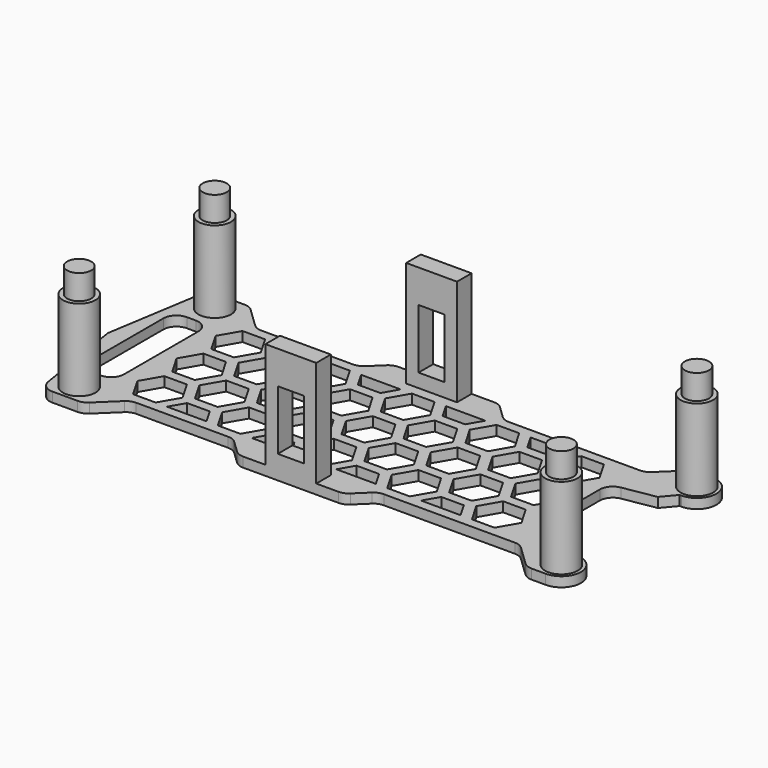
from build123d import *

# Parameters (mm, degrees)
F0_R         = 2.5
F0_W         = 5.3888335824
F0_H         = 18.2664785534
F1_DEPTH     = 1.5
F0_R_2       = 1.85
F2_DEPTH     = 14
F0_W_2       = 7.8
F0_H_2       = 2.8
F3_DEPTH     = 17.8
F4_W         = 3.9957887493
F4_H         = 9.1363643296
F5_DEPTH     = 32
F6_T4_DEPTH  = 11.8090227147
F6_S5_R      = 3
F6_T6_DEPTH  = 8
F6_T10_DEPTH = 11.8090227147
F6_S11_R     = 3
F6_T12_DEPTH = 8
F7_R         = 2


# Not quite as in the source:
# - a fillet or chamfer that OpenCascade refuses, or shapes differently, is made with other operations: its cross-section is extruded or revolved along the edge and cut away or added


with BuildPart() as f1:
    # F0 (on Top) → F1 (new body)
    with BuildSketch(Plane.XY):
        with BuildLine():
            Line((40, 8.2992520183), (40, 10))
            ThreePointArc((40, 10), (43, 13), (40, 16))
            Line((40, 16), (37.0306753963, 16))
            Line((37.0306753963, 16), (32.8572866916, 12))
            Line((32.8572866916, 12), (11.1427133083, 12))
            Line((11.1427133083, 12), (8.1170064975, 14.9))
            Line((8.1170064975, 14.9), (3.9, 14.9))
            Line((3.9, 14.9), (3.9, 12.1))
            Line((3.9, 12.1), (-3.9, 12.1))
            Line((-3.9, 12.1), (-3.9, 14.9))
            Line((-3.9, 14.9), (-8.1170064975, 14.9))
            Line((-8.1170064975, 14.9), (-11.1427133083, 12))
            Line((-11.1427133083, 12), (-26.8572866917, 12))
            Line((-26.8572866917, 12), (-31.0306753963, 16))
            Line((-31.0306753963, 16), (-37.4269299209, 16))
            Line((-37.4269299209, 16), (-40, 0))
            Line((-40, 0), (-37.4269299209, -16))
            Line((-37.4269299209, -16), (-31.0306753963, -16))
            Line((-31.0306753963, -16), (-26.8572866917, -12))
            Line((-26.8572866917, -12), (-11.1427133083, -12))
            Line((-11.1427133083, -12), (-8.1170064975, -14.9))
            Line((-8.1170064975, -14.9), (-3.9, -14.9))
            Line((-3.9, -14.9), (-3.9, -12.1))
            Line((-3.9, -12.1), (3.9, -12.1))
            Line((3.9, -12.1), (3.9, -14.9))
            Line((3.9, -14.9), (8.1170064975, -14.9))
            Line((8.1170064975, -14.9), (11.1427133083, -12))
            Line((11.1427133083, -12), (32.8572866916, -12))
            Line((32.8572866916, -12), (37.0306753963, -16))
            Line((37.0306753963, -16), (40, -16))
            ThreePointArc((40, -16), (43, -13), (40, -10))
            Line((40, -10), (40, -8.2992520183))
            Line((40, -8.2992520183), (31.389541924, -6.8237371743))
            Line((31.389541924, -6.8237371743), (31.389541924, 0))
            Line((31.389541924, 0), (31.389541924, 6.8237371743))
            Line((31.389541924, 6.8237371743), (40, 8.2992520183))
        make_face()
        with Locations((-34, -13)):
            Circle(F0_R, mode=Mode.SUBTRACT)
        Polygon((-16.4689110868, -10.5), (-22.5310889132, -10.5), (-21.2320508076, -8.25), (-17.7679491924, -8.25), align=None, mode=Mode.SUBTRACT)
        Polygon((-8.2320508076, -8.25), (-4.7679491924, -8.25), (-3.4689110868, -10.5), (-9.5310889132, -10.5), align=None, mode=Mode.SUBTRACT)
        Polygon((-24.2679491924, -10.5), (-27.7320508076, -10.5), (-29.4641016151, -7.5), (-27.7320508076, -4.5), (-24.2679491924, -4.5), (-22.5358983849, -7.5), align=None, mode=Mode.SUBTRACT)
        Polygon((-22.9641016151, -3.75), (-21.2320508076, -0.75), (-17.7679491924, -0.75), (-16.0358983849, -3.75), (-17.7679491924, -6.75), (-21.2320508076, -6.75), align=None, mode=Mode.SUBTRACT)
        Polygon((-11.2679491924, -10.5), (-14.7320508076, -10.5), (-16.4641016151, -7.5), (-14.7320508076, -4.5), (-11.2679491924, -4.5), (-9.5358983849, -7.5), align=None, mode=Mode.SUBTRACT)
        Polygon((-3.4641016151, -7.5), (-1.7320508076, -4.5), (1.7320508076, -4.5), (3.4641016151, -7.5), (1.7320508076, -10.5), (-1.7320508076, -10.5), align=None, mode=Mode.SUBTRACT)
        Polygon((-9.9641016151, -3.75), (-8.2320508076, -0.75), (-4.7679491924, -0.75), (-3.0358983849, -3.75), (-4.7679491924, -6.75), (-8.2320508076, -6.75), align=None, mode=Mode.SUBTRACT)
        Polygon((4.7679491924, -8.25), (8.2320508076, -8.25), (9.5310889132, -10.5), (3.4689110868, -10.5), align=None, mode=Mode.SUBTRACT)
        Polygon((17.7679491924, -8.25), (21.2320508076, -8.25), (22.5310889132, -10.5), (16.4689110868, -10.5), align=None, mode=Mode.SUBTRACT)
        with Locations((40, -13)):
            Circle(F0_R, mode=Mode.SUBTRACT)
        Polygon((11.2679491924, -10.5), (9.5358983849, -7.5), (11.2679491924, -4.5), (14.7320508076, -4.5), (16.4641016151, -7.5), (14.7320508076, -10.5), align=None, mode=Mode.SUBTRACT)
        Polygon((8.2320508076, -0.75), (9.9641016151, -3.75), (8.2320508076, -6.75), (4.7679491924, -6.75), (3.0358983849, -3.75), (4.7679491924, -0.75), align=None, mode=Mode.SUBTRACT)
        Polygon((16.0358983849, -3.75), (17.7679491924, -0.75), (21.2320508076, -0.75), (22.9641016151, -3.75), (21.2320508076, -6.75), (17.7679491924, -6.75), align=None, mode=Mode.SUBTRACT)
        Polygon((24.2679491924, -10.5), (22.5358983849, -7.5), (24.2679491924, -4.5), (27.7320508076, -4.5), (29.4641016151, -7.5), (27.7320508076, -10.5), align=None, mode=Mode.SUBTRACT)
        with Locations((-34.495420754, 0)):
            Rectangle(F0_W, F0_H, mode=Mode.SUBTRACT)
        Polygon((-27.7320508076, -3), (-29.4641016151, 0), (-27.7320508076, 3), (-24.2679491924, 3), (-22.5358983849, 0), (-24.2679491924, -3), align=None, mode=Mode.SUBTRACT)
        Polygon((-17.7679491924, 6.75), (-16.0358983849, 3.75), (-17.7679491924, 0.75), (-21.2320508076, 0.75), (-22.9641016151, 3.75), (-21.2320508076, 6.75), align=None, mode=Mode.SUBTRACT)
        Polygon((-29.4641016151, 7.5), (-27.7320508076, 10.5), (-24.2679491924, 10.5), (-22.5358983849, 7.5), (-24.2679491924, 4.5), (-27.7320508076, 4.5), align=None, mode=Mode.SUBTRACT)
        Polygon((-14.7320508076, -3), (-16.4641016151, 0), (-14.7320508076, 3), (-11.2679491924, 3), (-9.5358983849, 0), (-11.2679491924, -3), align=None, mode=Mode.SUBTRACT)
        Polygon((-3.4641016151, 0), (-1.7320508076, 3), (1.7320508076, 3), (3.4641016151, 0), (1.7320508076, -3), (-1.7320508076, -3), align=None, mode=Mode.SUBTRACT)
        Polygon((-4.7679491924, 6.75), (-3.0358983849, 3.75), (-4.7679491924, 0.75), (-8.2320508076, 0.75), (-9.9641016151, 3.75), (-8.2320508076, 6.75), align=None, mode=Mode.SUBTRACT)
        Polygon((-16.4641016151, 7.5), (-14.7320508076, 10.5), (-11.2679491924, 10.5), (-9.5358983849, 7.5), (-11.2679491924, 4.5), (-14.7320508076, 4.5), align=None, mode=Mode.SUBTRACT)
        Polygon((3.4641016151, 7.5), (1.7320508076, 4.5), (-1.7320508076, 4.5), (-3.4641016151, 7.5), (-1.7320508076, 10.5), (1.7320508076, 10.5), align=None, mode=Mode.SUBTRACT)
        Polygon((-21.2320508076, 8.25), (-22.5310889132, 10.5), (-16.4689110868, 10.5), (-17.7679491924, 8.25), align=None, mode=Mode.SUBTRACT)
        with Locations((-34, 13)):
            Circle(F0_R, mode=Mode.SUBTRACT)
        Polygon((-8.2320508076, 8.25), (-9.5310889132, 10.5), (-3.4689110868, 10.5), (-4.7679491924, 8.25), align=None, mode=Mode.SUBTRACT)
        Polygon((9.9641016151, 3.75), (8.2320508076, 0.75), (4.7679491924, 0.75), (3.0358983849, 3.75), (4.7679491924, 6.75), (8.2320508076, 6.75), align=None, mode=Mode.SUBTRACT)
        Polygon((16.4641016151, 0), (14.7320508076, -3), (11.2679491924, -3), (9.5358983849, 0), (11.2679491924, 3), (14.7320508076, 3), align=None, mode=Mode.SUBTRACT)
        Polygon((17.7679491924, 0.75), (16.0358983849, 3.75), (17.7679491924, 6.75), (21.2320508076, 6.75), (22.9641016151, 3.75), (21.2320508076, 0.75), align=None, mode=Mode.SUBTRACT)
        Polygon((11.2679491924, 4.5), (9.5358983849, 7.5), (11.2679491924, 10.5), (14.7320508076, 10.5), (16.4641016151, 7.5), (14.7320508076, 4.5), align=None, mode=Mode.SUBTRACT)
        Polygon((29.4641016151, 0), (27.7320508076, -3), (24.2679491924, -3), (22.5358983849, 0), (24.2679491924, 3), (27.7320508076, 3), align=None, mode=Mode.SUBTRACT)
        Polygon((24.2679491924, 4.5), (22.5358983849, 7.5), (24.2679491924, 10.5), (27.7320508076, 10.5), (29.4641016151, 7.5), (27.7320508076, 4.5), align=None, mode=Mode.SUBTRACT)
        Polygon((4.7679491924, 8.25), (3.4689110868, 10.5), (9.5310889132, 10.5), (8.2320508076, 8.25), align=None, mode=Mode.SUBTRACT)
        Polygon((17.7679491924, 8.25), (16.4689110868, 10.5), (22.5310889132, 10.5), (21.2320508076, 8.25), align=None, mode=Mode.SUBTRACT)
        with Locations((40, 13)):
            Circle(F0_R, mode=Mode.SUBTRACT)
    extrude(amount=F1_DEPTH)

    # F0 (on Top) → F2 (join)
    with BuildSketch(Plane.XY):
        with Locations((40, -13)):
            Circle(F0_R)
        with Locations((40, -13)):
            Circle(F0_R_2, mode=Mode.SUBTRACT)
        with Locations((40, 13)):
            Circle(F0_R)
        with Locations((40, 13)):
            Circle(F0_R_2, mode=Mode.SUBTRACT)
        with Locations((-34, -13)):
            Circle(F0_R)
        with Locations((-34, -13)):
            Circle(F0_R_2, mode=Mode.SUBTRACT)
        with Locations((-34, 13)):
            Circle(F0_R)
        with Locations((-34, 13)):
            Circle(F0_R_2, mode=Mode.SUBTRACT)
    extrude(amount=F2_DEPTH)

    # F0 (on Top) → F3 (join)
    with BuildSketch(Plane.XY):
        with Locations((-34, -13)):
            Circle(F0_R_2)
        with Locations((-34, 13)):
            Circle(F0_R_2)
        with Locations((40, 13)):
            Circle(F0_R_2)
        with Locations((40, -13)):
            Circle(F0_R_2)
        with Locations((0, 13.5)):
            Rectangle(F0_W_2, F0_H_2)
        with Locations((0, -13.5)):
            Rectangle(F0_W_2, F0_H_2)
    extrude(amount=F3_DEPTH)

    # F4 (on face) → F5 (cut)
    with BuildSketch(Plane.XZ.offset(14.9)):
        with Locations((0, 8.1683266908)):
            Rectangle(F4_W, F4_H)
    extrude(amount=-F5_DEPTH, mode=Mode.SUBTRACT)

    # F6: chamfer of 2 on 2 edges, made by hand


with BuildPart() as f6_tool2:
    # F6_s3 → F6_t4 (new body)
    with BuildSketch(Plane.XY.offset(-5.1545113574)):
        Polygon((38.0287340033, 7.9614497534), (40, 10.2992520183), (40, 8.2992520183), align=None)
    extrude(amount=F6_T4_DEPTH)

    # F6_s5 → F6_t6 (cut, symmetric)
    with BuildSketch(Plane.XY.offset(0.7)):
        with Locations((40, 13)):
            Circle(F6_S5_R)
    extrude(amount=F6_T6_DEPTH, both=True, mode=Mode.SUBTRACT)


with BuildPart() as f1_1:
    add(f1.part)

    # F6_t1: cut F6_tool2
    add(f6_tool2.part, mode=Mode.SUBTRACT)


with BuildPart() as f6_tool8:
    # F6_s9 → F6_t10 (new body)
    with BuildSketch(Plane.XY.offset(-5.1545113574)):
        Polygon((40, -10.2992520183), (38.0287340033, -7.9614497534), (40, -8.2992520183), align=None)
    extrude(amount=F6_T10_DEPTH)

    # F6_s11 → F6_t12 (cut, symmetric)
    with BuildSketch(Plane.XY.offset(0.7)):
        with Locations((40, -13)):
            Circle(F6_S11_R)
    extrude(amount=F6_T12_DEPTH, both=True, mode=Mode.SUBTRACT)


with BuildPart() as f1_2:
    add(f1_1.part)

    # F6_t7: cut F6_tool8
    add(f6_tool8.part, mode=Mode.SUBTRACT)

    # F7
    f7_edges = [f1_2.edges().sort_by_distance(p)[0] for p in [
        (31.389542, -6.823737, 0.75),
        (31.389542, 6.823737, 0.75),
        (-31.801004, 9.133239, 0.75),
        (-37.189838, 9.133239, 0.75),
        (-37.189838, -9.133239, 0.75),
        (-31.801004, -9.133239, 0.75),
        (-37.42693, 16, 0.75),
        (-37.42693, -16, 0.75),
        (-31.030675, 16, 0.75),
        (-26.857287, 12, 0.75),
        (-11.142713, 12, 0.75),
        (-8.117006, 14.9, 0.75),
        (8.117006, 14.9, 0.75),
        (11.142713, 12, 0.75),
        (32.857287, 12, 0.75),
        (37.030675, 16, 0.75),
        (37.030675, -16, 0.75),
        (32.857287, -12, 0.75),
        (11.142713, -12, 0.75),
        (8.117006, -14.9, 0.75),
        (-8.117006, -14.9, 0.75),
        (-11.142713, -12, 0.75),
        (-26.857287, -12, 0.75),
        (-31.030675, -16, 0.75),
    ]]
    fillet(f7_edges, radius=F7_R)


solid = f1_2.part
